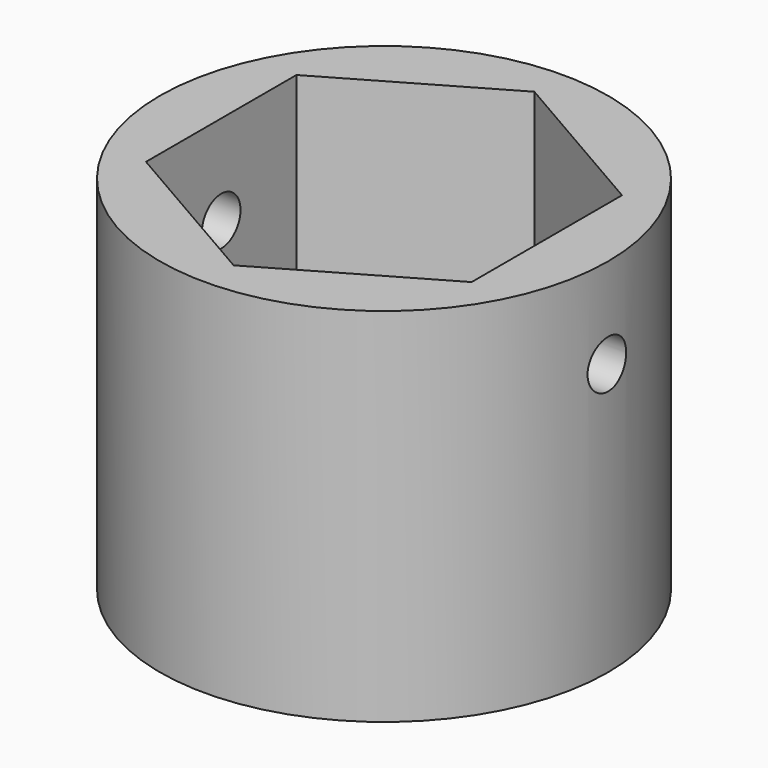
from build123d import *

# Parameters (mm, degrees)
F0_R          = 18.5884572681
F1_DEPTH      = 30
F2_R          = 2
F3_DEPTH      = 5.0894572681
F3_DEPTH_BACK = 32.0894572681


# Not quite as in the source:
# - a feature names something its author has since deleted; it is built from what else it names


with BuildPart() as f1:
    # F0 (on Top) → F1 (new body)
    with BuildSketch(Plane.XY):
        Circle(F0_R)
        Polygon((0, 15.5884572681), (13.5, 7.7942286341), (13.5, -7.7942286341), (0, -15.5884572681), (-13.5, -7.7942286341), (-13.5, 7.7942286341), align=None, mode=Mode.SUBTRACT)
    extrude(amount=F1_DEPTH)

    # F2 (on face) → F3 (cut, two sides)
    with BuildSketch(Plane.YZ.offset(-13.5)) as f3_sk:
        with Locations((0, 22.5)):
            Circle(F2_R)
    extrude(amount=-F3_DEPTH, mode=Mode.SUBTRACT)
    extrude(f3_sk.sketch, amount=F3_DEPTH_BACK, mode=Mode.SUBTRACT)


solid = f1.part
